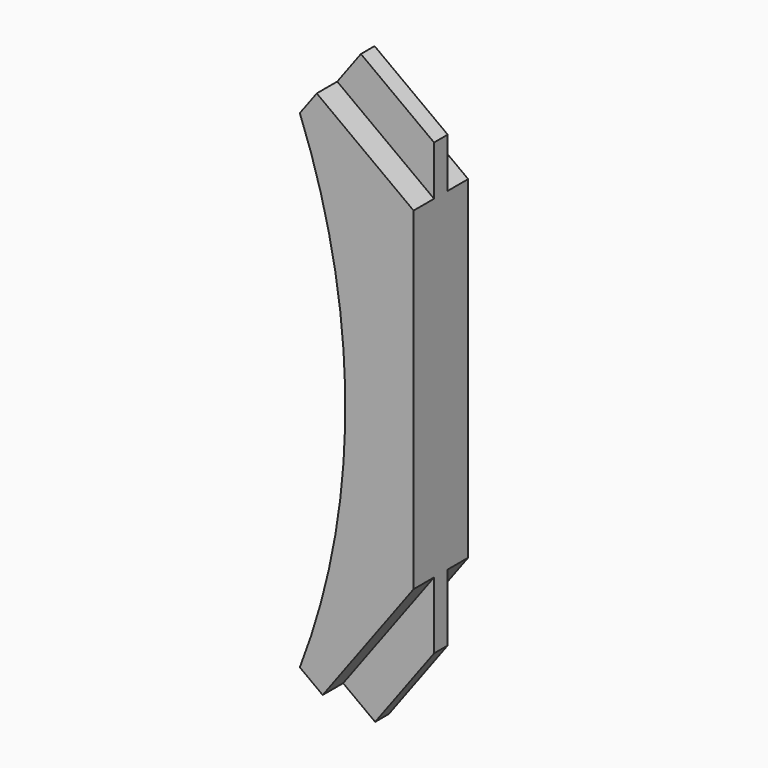
from build123d import *

# Parameters (mm, degrees)
F1_DEPTH = 76.2
F2_DEPTH = 19.05


# Not quite as in the source:
# - a feature names something its author has since deleted; it is built from what else it names


with BuildPart() as f1:
    # F0 (on Front) → F1 (new body, symmetric)
    with BuildSketch(Plane.XZ):
        with BuildLine():
            Line((127, 339.2728872618), (-127, 527.42103541))
            ThreePointArc((-127, 527.42103541), (-25.4, -17.4321152174), (-127, -562.2852658447))
            Line((-127, -562.2852658447), (127, -219.3852658447))
            Line((127, -219.3852658447), (127, 339.2728872618))
        make_face()
        Polygon((127, -219.3852658447), (-127, -562.2852658447), (-96.3844709336, -584.9634355236), (127, -283.3943997633), align=None)
        Polygon((-104.3218303212, 558.0365644764), (-127, 527.42103541), (127, 339.2728872618), (127, 386.6870605348), align=None)
        Polygon((127, -283.3943997633), (-96.3844709336, -584.9634355236), (-75.9741182226, -600.0822153095), (127, -326.067155709), align=None)
        Polygon((-89.2030505353, 578.4469171874), (-104.3218303212, 558.0365644764), (127, 386.6870605348), (127, 418.2965093835), align=None)
    extrude(amount=F1_DEPTH, both=True)

    # F0 (on Front) → F2 (join, symmetric)
    with BuildSketch(Plane.XZ):
        Polygon((127, -326.067155709), (-75.9741182226, -600.0822153095), (-4.5378837343, -652.9979445601), (127, -475.4218015188), align=None)
        Polygon((127, 418.2965093835), (127, 528.9295803538), (-36.2873212846, 649.8831516757), (-89.2030505353, 578.4469171874), align=None)
    extrude(amount=F2_DEPTH, both=True)


solid = f1.part
